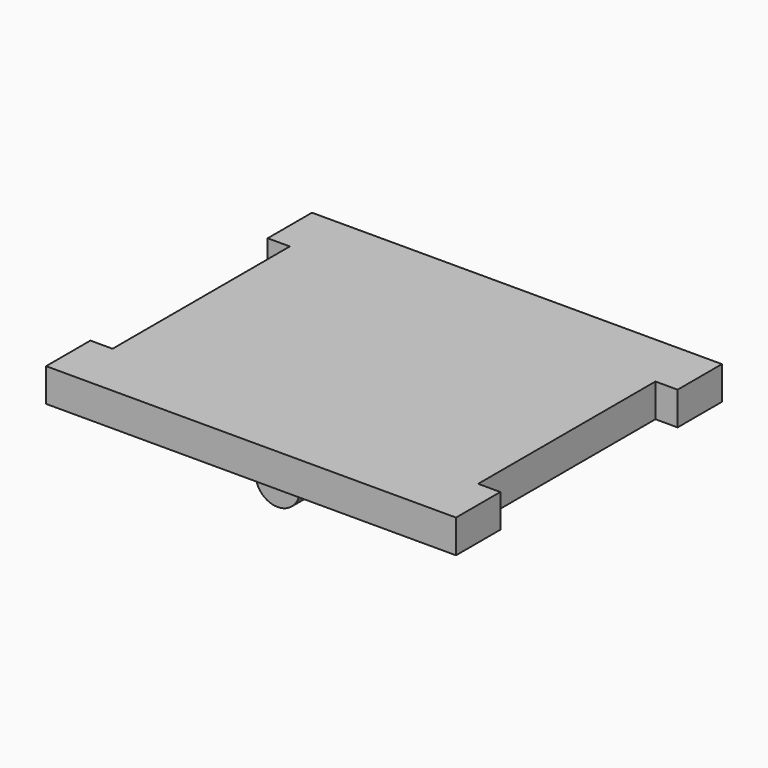
from build123d import *

# Parameters (mm, degrees)
F0_W     = 2
F0_H     = 1.5
F0_H_2   = 20
F0_W_2   = 11
F0_W_3   = 7
F1_DEPTH = 3
F3_DEPTH = 26.5
F5_R     = 2
F6_DEPTH = 27
F7_R     = 0.75
F8_DEPTH = 0.5
F9_R     = 0.49999


# Not quite as in the source:
# - a fillet or chamfer is up to 0.001 mm smaller than in the source, because OpenCascade refuses the exact size


with BuildPart() as f1:
    # F0 (on Top) → F1 (new body)
    with BuildSketch(Plane.XY):
        Polygon((-1.7407407407, 9.2222222222), (5.2592592593, 9.2222222222), (16.2592592593, 9.2222222222), (16.2592592593, 10.7222222222), (18.2592592593, 10.7222222222), (18.2592592593, 9.2222222222), (20.2592592593, 9.2222222222), (20.2592592593, 14.2222222222), (-16.7407407407, 14.2222222222), (-16.7407407407, 9.2222222222), (-14.7407407407, 9.2222222222), (-14.7407407407, 10.7222222222), (-12.7407407407, 10.7222222222), (-12.7407407407, 9.2222222222), align=None)
        Polygon((16.2592592593, -10.7777777778), (5.2592592593, -10.7777777778), (-1.7407407407, -10.7777777778), (-12.7407407407, -10.7777777778), (-12.7407407407, -12.2777777778), (-14.7407407407, -12.2777777778), (-14.7407407407, -10.7777777778), (-16.7407407407, -10.7777777778), (-16.7407407407, -15.7777777778), (20.2592592593, -15.7777777778), (20.2592592593, -10.7777777778), (18.2592592593, -10.7777777778), (18.2592592593, -12.2777777778), (16.2592592593, -12.2777777778), align=None)
        with Locations((17.2592592593, 9.9722222222)):
            Rectangle(F0_W, F0_H)
        with Locations((17.2592592593, -0.7777777778)):
            Rectangle(F0_W, F0_H_2)
        with Locations((-13.7407407407, -0.7777777778)):
            Rectangle(F0_W, F0_H_2)
        with Locations((-13.7407407407, 9.9722222222)):
            Rectangle(F0_W, F0_H)
        with Locations((17.2592592593, -11.5277777778)):
            Rectangle(F0_W, F0_H)
        with Locations((-13.7407407407, -11.5277777778)):
            Rectangle(F0_W, F0_H)
        with Locations((-7.2407407407, -0.7777777778)):
            Rectangle(F0_W_2, F0_H_2)
        with Locations((1.7592592593, -0.7777777778)):
            Rectangle(F0_W_3, F0_H_2)
        with Locations((10.7592592593, -0.7777777778)):
            Rectangle(F0_W_2, F0_H_2)
    extrude(amount=F1_DEPTH)

    # F5 (on face) → F6 (join)
    with BuildSketch(Plane(origin=(0, 14.2222222222, 0), x_dir=(-1, 0, 0), z_dir=(0, 1, 0))):
        with Locations((-1.7592592593, -1.4)):
            Circle(F5_R)
    extrude(amount=-F6_DEPTH)

    # F7 (on face) → F8 (join)
    with BuildSketch(Plane(origin=(0, 0, 0), x_dir=(1, 0, 0), z_dir=(0, 0, -1))):
        with Locations((-7.2407407407, 13.2777777778)):
            Circle(F7_R)
        with Locations((10.7592592593, 13.2777777778)):
            Circle(F7_R)
    extrude(amount=F8_DEPTH)

    # F9 (radius 0.5 in the source; OpenCascade refuses exactly that, so slightly less here)
    f9_edges = [f1.edges().sort_by_distance(p)[0] for p in [
        (10.009259, -13.277778, -0.5),
        (-7.990741, -13.277778, -0.5),
    ]]
    fillet(f9_edges, radius=F9_R)


with BuildPart() as f3:
    # F2 (on face) → F3 (new body)
    with BuildSketch(Plane(origin=(0, 14.2222222222, 0), x_dir=(-1, 0, 0), z_dir=(0, 1, 0))):
        with BuildLine():
            ThreePointArc((-1.3930631716, 0), (-0.7580650487, -3.223722123), (1.975, -1.4))
            ThreePointArc((1.975, -1.4), (1.823722123, -0.6419349513), (1.3930631716, 0))
            Line((1.3930631716, 0), (-1.3930631716, 0))
        make_face()
    extrude(amount=-F3_DEPTH)


solid = f1.part
